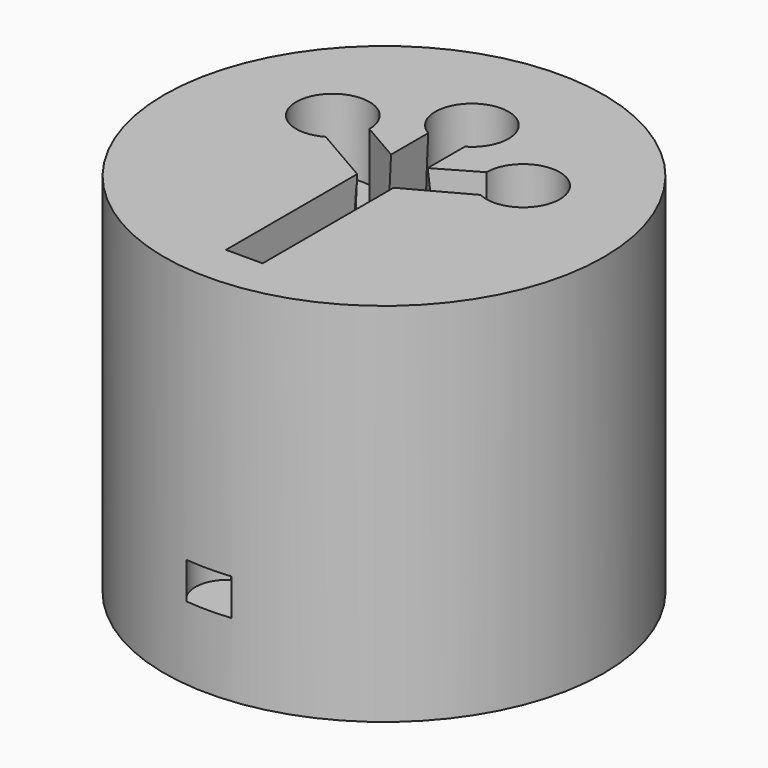
from build123d import *

# Parameters (mm, degrees)
F0_R                   = 76.2
F1_DEPTH               = 127
F3_R                   = 11.2611691567
F4_DEPTH               = 12.7
F7_DEPTH               = 25.4
F8_DEPTH               = 25.4
DRAFT_F8_DRAFTED_ANGLE = -5
F9_DEPTH               = 101.6


# Not quite as in the source:
# - an extrude with a draft is written as a straight extrude whose walls are then drafted


with BuildPart() as f1:
    # F0 (on Top) → F1 (new body)
    with BuildSketch(Plane.XY):
        Circle(F0_R)
    extrude(amount=F1_DEPTH)

    # F3 (on offset) → F4 (cut)
    with BuildSketch(Plane.XY.offset(25.4)):
        with Locations((0, -67.7085220814)):
            Circle(F3_R)
    extrude(amount=F4_DEPTH, mode=Mode.SUBTRACT)

    # F6 (on offset) → F7 (cut)
    with BuildSketch(Plane.XY.offset(127)):
        with BuildLine():
            Line((6.35, 38.1), (6.35, 27.1014773719))
            ThreePointArc((6.35, 27.1014773719), (10.9985226281, 31.75), (12.7, 38.1))
            ThreePointArc((12.7, 38.1), (-6.35, 49.0985226281), (-6.35, 27.1014773719))
            Line((-6.35, 27.1014773719), (-6.35, 38.1))
            Line((-6.35, 38.1), (6.35, 38.1))
        make_face()
        with BuildLine():
            ThreePointArc((-6.35, 27.1014773719), (0, 25.4), (6.35, 27.1014773719))
            Line((6.35, 27.1014773719), (6.35, 38.1))
            Line((6.35, 38.1), (-6.35, 38.1))
            Line((-6.35, 38.1), (-6.35, 27.1014773719))
        make_face()
        with BuildLine():
            Line((-29.8205678842, 24.549261314), (-20.2955678842, 19.05))
            ThreePointArc((-20.2955678842, 19.05), (-43.9940905122, 25.4), (-26.6455678842, 8.0514773719))
            Line((-26.6455678842, 8.0514773719), (-36.1705678842, 13.550738686))
            Line((-36.1705678842, 13.550738686), (-32.9955678842, 19.05))
            Line((-32.9955678842, 19.05), (-29.8205678842, 24.549261314))
        make_face()
        with BuildLine():
            ThreePointArc((45.6955678842, 19.05), (32.9955678842, 31.75), (20.2955678842, 19.05))
            Line((20.2955678842, 19.05), (29.8205678842, 24.549261314))
            Line((29.8205678842, 24.549261314), (32.9955678842, 19.05))
            Line((32.9955678842, 19.05), (36.6617420935, 12.7))
            Line((36.6617420935, 12.7), (27.3832685469, 7.6573665841))
            ThreePointArc((27.3832685469, 7.6573665841), (39.7042860336, 8.2665357704), (45.6955678842, 19.05))
        make_face()
        with BuildLine():
            Line((29.8205678842, 24.549261314), (20.2955678842, 19.05))
            ThreePointArc((20.2955678842, 19.05), (22.2121036546, 12.3412818506), (27.3832685469, 7.6573665841))
            Line((27.3832685469, 7.6573665841), (36.6617420935, 12.7))
            Line((36.6617420935, 12.7), (32.9955678842, 19.05))
            Line((32.9955678842, 19.05), (29.8205678842, 24.549261314))
        make_face()
        with BuildLine():
            ThreePointArc((-26.6455678842, 8.0514773719), (-21.9970452561, 12.7), (-20.2955678842, 19.05))
            Line((-20.2955678842, 19.05), (-29.8205678842, 24.549261314))
            Line((-29.8205678842, 24.549261314), (-32.9955678842, 19.05))
            Line((-32.9955678842, 19.05), (-36.1705678842, 13.550738686))
            Line((-36.1705678842, 13.550738686), (-26.6455678842, 8.0514773719))
        make_face()
        with BuildLine():
            Line((-6.35, -3.6661742094), (-6.35, 0))
            Line((-6.35, 0), (-6.35, 10.9985226281))
            Line((-6.35, 10.9985226281), (-20.2955678842, 19.05))
            ThreePointArc((-20.2955678842, 19.05), (-21.9970452561, 12.7), (-26.6455678842, 8.0514773719))
            Line((-26.6455678842, 8.0514773719), (-6.35, -3.6661742094))
        make_face()
        Polygon((-6.35, 0), (0, 0), (-3.175, 5.499261314), (0, 7.3323484187), (-6.35, 10.9985226281), align=None)
        Polygon((-3.175, 5.499261314), (0, 0), (3.175, 5.499261314), (0, 7.3323484187), align=None)
        Polygon((-3.175, -5.499261314), (0, 0), (-6.35, 0), (-6.35, -3.6661742094), align=None)
        with BuildLine():
            Line((6.35, 10.9985226281), (6.35, 0))
            Line((6.35, 0), (6.35, -3.7737230544))
            Line((6.35, -3.7737230544), (27.3832685469, 7.6573665841))
            ThreePointArc((27.3832685469, 7.6573665841), (22.2121036546, 12.3412818506), (20.2955678842, 19.05))
            Line((20.2955678842, 19.05), (6.35, 10.9985226281))
        make_face()
        Polygon((0, 0), (6.35, 0), (6.35, 10.9985226281), (0, 7.3323484187), (3.175, 5.499261314), align=None)
        Polygon((6.35, -3.7737230544), (6.35, 0), (0, 0), (3.175, -5.499261314), align=None)
    extrude(amount=-F7_DEPTH, mode=Mode.SUBTRACT)


with BuildPart() as f8_drafted:
    # F6 (on offset) → F8 (new body)
    with BuildSketch(Plane.XY.offset(127)):
        Polygon((-6.35, 0), (0, 0), (-3.175, 5.499261314), (0, 7.3323484187), (-6.35, 10.9985226281), align=None)
        with BuildLine():
            Line((0, 7.3323484187), (6.35, 10.9985226281))
            Line((6.35, 10.9985226281), (6.35, 27.1014773719))
            ThreePointArc((6.35, 27.1014773719), (0, 25.4), (-6.35, 27.1014773719))
            Line((-6.35, 27.1014773719), (-6.35, 10.9985226281))
            Line((-6.35, 10.9985226281), (0, 7.3323484187))
        make_face()
        Polygon((-3.175, -5.499261314), (0, 0), (-6.35, 0), (-6.35, -3.6661742094), align=None)
        Polygon((-3.175, 5.499261314), (0, 0), (3.175, 5.499261314), (0, 7.3323484187), align=None)
        Polygon((6.35, -3.7737230544), (6.35, 0), (0, 0), (3.175, -5.499261314), align=None)
        Polygon((0, 0), (6.35, 0), (6.35, 10.9985226281), (0, 7.3323484187), (3.175, 5.499261314), align=None)
    extrude(amount=-F8_DEPTH)

    # draft_F8_drafted
    draft_f8_drafted_walls = [f8_drafted.faces().sort_by_distance(p)[0] for p in [
        (0, 25.4, 110.0666666667),
        (-6.35, 11.7176515813, 110.0666666667),
        (-4.7625, -4.5827177617, 110.0666666667),
        (-1.5875, -2.749630657, 110.0666666667),
        (1.5875, -2.749630657, 110.0666666667),
        (4.7625, -4.6364921842, 110.0666666667),
        (6.35, 11.6638771588, 110.0666666667),
    ]]
    draft(draft_f8_drafted_walls, neutral_plane=Plane(origin=(0, 0, 127), x_dir=(1, 0, 0), z_dir=(0, 0, -1)), angle=DRAFT_F8_DRAFTED_ANGLE)


with BuildPart() as f1_1:
    add(f1.part)

    # join_F8_drafted: cut F8_drafted
    add(f8_drafted.part, mode=Mode.SUBTRACT)

    # F6 (on offset) → F9 (cut)
    with BuildSketch(Plane.XY.offset(127)):
        Polygon((3.175, -5.499261314), (0, 0), (-3.175, -5.499261314), (-6.35, -3.6661742094), (-6.35, -60.5426877737), (6.35, -60.5426877737), (6.35, -3.7737230544), align=None)
        Polygon((-3.175, -5.499261314), (0, 0), (-6.35, 0), (-6.35, -3.6661742094), align=None)
        Polygon((6.35, -3.7737230544), (6.35, 0), (0, 0), (3.175, -5.499261314), align=None)
    extrude(amount=-F9_DEPTH, mode=Mode.SUBTRACT)


solid = f1_1.part
